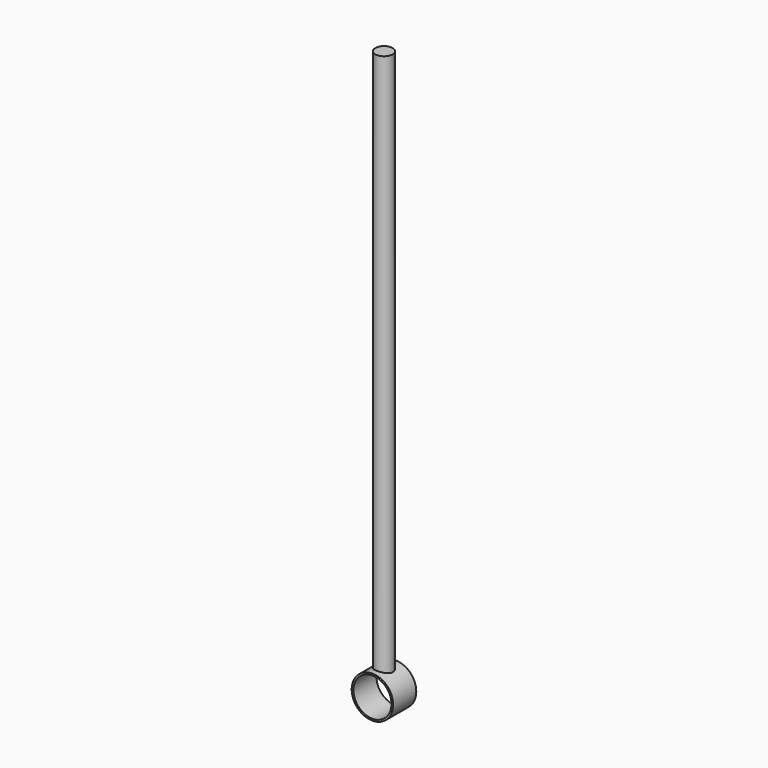
from build123d import *

# Parameters (mm, degrees)
F0_R          = 18
F0_R_2        = 16.5
F1_DEPTH      = 25
F2_R          = 7.5
F3_DEPTH      = 488
F4_END_RADIUS = 16.5
F3_FACE_R     = 7.5
F4_REACH      = 509.2142035356


with BuildPart() as f1:
    # F0 (on Front) → F1 (new body)
    with BuildSketch(Plane.XZ):
        Circle(F0_R)
        Circle(F0_R_2, mode=Mode.SUBTRACT)
    extrude(amount=F1_DEPTH)

    # F2 (on Top) → F3 (join)
    with BuildSketch(Plane.XY):
        with Locations((0, -12.5)):
            Circle(F2_R)
    extrude(amount=F3_DEPTH)

    f4_end = (Plane.ZX.offset(-12.5) * Cylinder(F4_END_RADIUS, 2034.2177557588, mode=Mode.PRIVATE)).faces().sort_by_distance((-16.5, -12.5, 0))[0]
    # F3_face (on face) → F4 (cut, up to the whole of a round face its end follows)
    with BuildSketch(Plane(origin=(0, -12.5, 0), x_dir=(1, 0, 0), z_dir=(0, 0, -1))):
        Circle(F3_FACE_R)
    f4_long = extrude(amount=-F4_REACH, mode=Mode.PRIVATE)
    add(split(f4_long, bisect_by=f4_end, keep=Keep.BOTTOM, mode=Mode.PRIVATE), mode=Mode.SUBTRACT)


solid = f1.part
